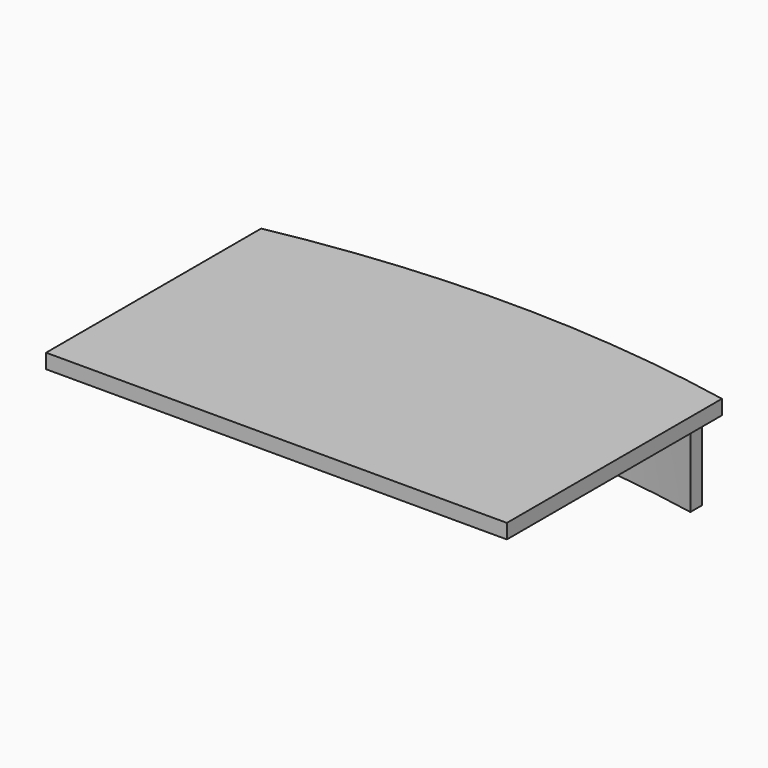
from build123d import *

# Parameters (mm, degrees)
F1_DEPTH = 19
F3_DEPTH = 100


# Not quite as in the source:
# - a feature of the source that left no trace in its solid (it failed there, or was rolled back) is left out


with BuildPart() as f1:
    # F0 (on Top) → F1 (new body)
    with BuildSketch(Plane.XY):
        with BuildLine():
            Line((-300, -175), (300, -175))
            Line((300, -175), (300, 175))
            ThreePointArc((300, 175), (0, 204.3093674254), (-300, 175))
            Line((-300, 175), (-300, -175))
        make_face()
    extrude(amount=F1_DEPTH)

    # F2 (on face) → F3 (join)
    with BuildSketch(Plane(origin=(0, 0, 0), x_dir=(1, 0, 0), z_dir=(0, 0, -1))):
        with BuildLine():
            Line((-288, -138.6273926478), (-288, -157.9772163868))
            ThreePointArc((-288, -157.9772163868), (0, -185.3093674254), (288, -157.9772163868))
            Line((288, -157.9772163868), (288, -138.6273926478))
            ThreePointArc((288, -138.6273926478), (0, -166.3093674254), (-288, -138.6273926478))
        make_face()
    extrude(amount=F3_DEPTH)


solid = f1.part
